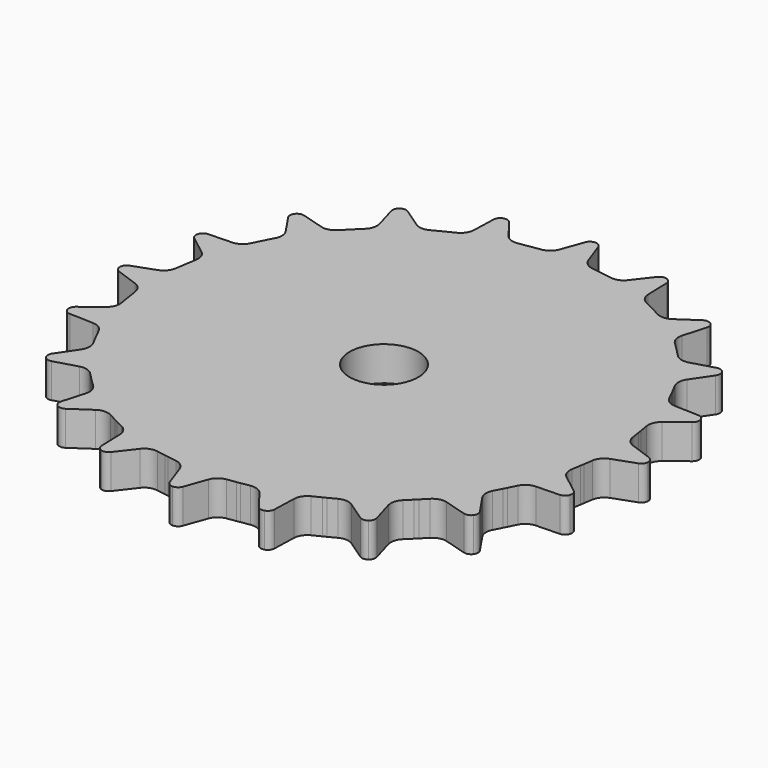
from build123d import *

# Parameters (mm, degrees)
F1_DEPTH        = 1
F1_COPIES_COUNT = 20
F3_R            = 1
F4_DEPTH        = 1.001


# Not quite as in the source:
# - a feature of the source that left no trace in its solid (it failed there, or was rolled back) is left out
# - a pattern or mirror of a feature is missing from the dataset's text; its kind, count and spacing are read off the source's solid


with BuildPart() as f1:
    # F0 (on Top) → F1 (new body)
    with BuildSketch(Plane.XY):
        with BuildLine():
            Line((0, 7.685), (0, 7.285))
            ThreePointArc((0, 7.285), (0.1414213562, 7.3435786438), (0.2, 7.485))
            ThreePointArc((0.2, 7.485), (0.1970321115, 7.5193270599), (0.1882165296, 7.552635331))
            ThreePointArc((0.1882165296, 7.552635331), (0.1150498453, 7.648595639), (0, 7.685))
        make_face()
        with BuildLine():
            ThreePointArc((-0.1882165296, 7.552635331), (-0.163595639, 7.3699501547), (0, 7.285))
            Line((0, 7.285), (0, 7.685))
            ThreePointArc((0, 7.685), (-0.1150498453, 7.648595639), (-0.1882165296, 7.552635331))
        make_face()
        with BuildLine():
            Line((-0.7361660383, 6.6494735036), (-0.9944369312, 6.6106217703))
            ThreePointArc((-0.9944369312, 6.6106217703), (-0.4986072932, 6.6663795097), (0, 6.685))
            Line((0, 6.685), (0, 7.285))
            ThreePointArc((0, 7.285), (-0.163595639, 7.3699501547), (-0.1882165296, 7.552635331))
            Line((-0.1882165296, 7.552635331), (-0.4192355629, 6.9097523866))
            ThreePointArc((-0.4192355629, 6.9097523866), (-0.5418059714, 6.7359053452), (-0.7361660383, 6.6494735036))
        make_face()
        with BuildLine():
            ThreePointArc((0, 6.685), (0.4986072932, 6.6663795097), (0.9944369312, 6.6106217703))
            Line((0.9944369312, 6.6106217703), (0.7361660383, 6.6494735036))
            ThreePointArc((0.7361660383, 6.6494735036), (0.5418059714, 6.7359053452), (0.4192355629, 6.9097523866))
            Line((0.4192355629, 6.9097523866), (0.1882165296, 7.552635331))
            ThreePointArc((0.1882165296, 7.552635331), (0.1970321115, 7.5193270599), (0.2, 7.485))
            ThreePointArc((0.2, 7.485), (0.1414213562, 7.3435786438), (0, 7.285))
            Line((0, 7.285), (0, 6.685))
        make_face()
        with BuildLine():
            ThreePointArc((-0.9944369312, 6.6106217703), (-4.3612735591, -5.0664107554), (6.685, 0))
            ThreePointArc((6.685, 0), (5.0664107554, 4.3612735591), (0.9944369312, 6.6106217703))
            ThreePointArc((0.9944369312, 6.6106217703), (0.4986072932, 6.6663795097), (0, 6.685))
            ThreePointArc((0, 6.685), (-0.4986072932, 6.6663795097), (-0.9944369312, 6.6106217703))
        make_face()
    extrude(amount=F1_DEPTH)

    # F1_copies: F1 ×20 about axis
    f1_copies_axis = Axis((0, 0, 0), (0, 0, 1))


with BuildPart() as f1_1:
    add(f1.part)
    for i in range(1, F1_COPIES_COUNT):
        add(f1.part.rotate(f1_copies_axis, i * 360 / F1_COPIES_COUNT))

    # F3 (on face) → F4 (cut, through all)
    with BuildSketch(Plane.XY.offset(1)):
        Circle(F3_R)
    extrude(amount=-F4_DEPTH, mode=Mode.SUBTRACT)


solid = f1_1.part
